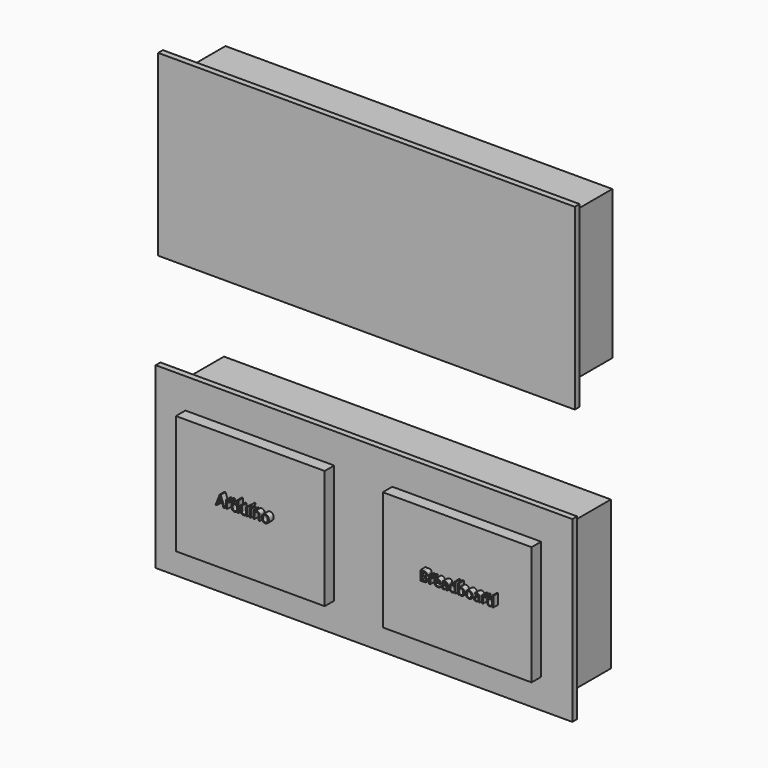
from build123d import *

# Parameters (mm, degrees)
F0_W           = 177.8
F0_H           = 76.2
F1_DEPTH       = 2.54
F2_W           = 63.5
F2_H           = 50.8
F3_DEPTH       = 5.08
F4_TEXT_SIZE   = 6.1658288663
F4_TEXT_SIZE_2 = 5.7428143919
F5_DEPTH       = 2.54
F6_W           = 165.1
F6_H           = 63.5
F7_DEPTH       = 25.4
F8_TEXT_SIZE   = 29.7080673691
F9_DEPTH       = 2.54
F10_W          = 177.8
F10_H          = 76.2
F11_DEPTH      = 2.54
F12_W          = 165.1
F12_H          = 63.5
F13_DEPTH      = 25.4
F14_TEXT_SIZE  = 36.0313285556
F15_DEPTH      = 2.54
F16_DEPTH      = 25.4


# Not quite as in the source:
# - Text() gives the source's letters only with a copy of the font that has no kerning and outlines rounded to 1/6400 em; it was checked with that copy


with BuildPart() as f1:
    # F0 (on Front) → F1 (new body)
    with BuildSketch(Plane.XZ):
        with Locations((0.191677545, 21.1522702593)):
            Rectangle(F0_W, F0_H)
    extrude(amount=F1_DEPTH)

    # F2 (on face) → F3 (join)
    with BuildSketch(Plane.XZ.offset(2.54)):
        with Locations((-44.258322455, 20.9469393546)):
            Rectangle(F2_W, F2_H)
        with Locations((44.0236674622, 21.0317056626)):
            Rectangle(F2_W, F2_H)
    extrude(amount=F3_DEPTH)

    # F4 (on face) → F5 (join)
    with BuildSketch(Plane.XZ.offset(7.62)):
        with Locations((-57.0269525051, 20.202929154)):
            Text('Arduino', F4_TEXT_SIZE, font='Open Sans', text_align=(TextAlign.LEFT, TextAlign.BOTTOM))
        with Locations((29.8993270844, 20.1223604381)):
            Text('Breadboard', F4_TEXT_SIZE_2, font='Open Sans', text_align=(TextAlign.LEFT, TextAlign.BOTTOM))
    extrude(amount=F5_DEPTH)

    # F6 (on face) → F7 (join)
    with BuildSketch(Plane(origin=(0, 0, 0), x_dir=(-1, 0, 0), z_dir=(0, 1, 0))):
        with Locations((-0.6299052119, 21.5918692648)):
            Rectangle(F6_W, F6_H)
    extrude(amount=F7_DEPTH)

    # F8 (on face) → F9 (join)
    with BuildSketch(Plane(origin=(0, 25.4, 0), x_dir=(-1, 0, 0), z_dir=(0, 1, 0))):
        with Locations((-42.1641431749, 13.6208720505)):
            Text('Foam', F8_TEXT_SIZE, font='Open Sans', text_align=(TextAlign.LEFT, TextAlign.BOTTOM))
    extrude(amount=F9_DEPTH)

    # F6 (on face) → F16 (join)
    with BuildSketch(Plane(origin=(0, 0, 0), x_dir=(-1, 0, 0), z_dir=(0, 1, 0))):
        with Locations((-0.6299052119, 21.5918692648)):
            Rectangle(F6_W, F6_H)
    extrude(amount=F16_DEPTH)


with BuildPart() as f11:
    # F10 (on Front) → F11 (new body)
    with BuildSketch(Plane.XZ):
        with Locations((1.2485608459, 138.8317614685)):
            Rectangle(F10_W, F10_H)
    extrude(amount=F11_DEPTH)

    # F12 (on face) → F13 (join)
    with BuildSketch(Plane(origin=(0, 0, 0), x_dir=(-1, 0, 0), z_dir=(0, 1, 0))):
        with Locations((-1.2727487564, 138.4477530718)):
            Rectangle(F12_W, F12_H)
    extrude(amount=F13_DEPTH)

    # F14 (on face) → F15 (join)
    with BuildSketch(Plane(origin=(0, 25.4, 0), x_dir=(-1, 0, 0), z_dir=(0, 1, 0))):
        with Locations((-53.1239584088, 124.9763593078)):
            Text('Foam', F14_TEXT_SIZE, font='Open Sans', text_align=(TextAlign.LEFT, TextAlign.BOTTOM))
    extrude(amount=F15_DEPTH)


solid = Compound([f1.part, f11.part])
